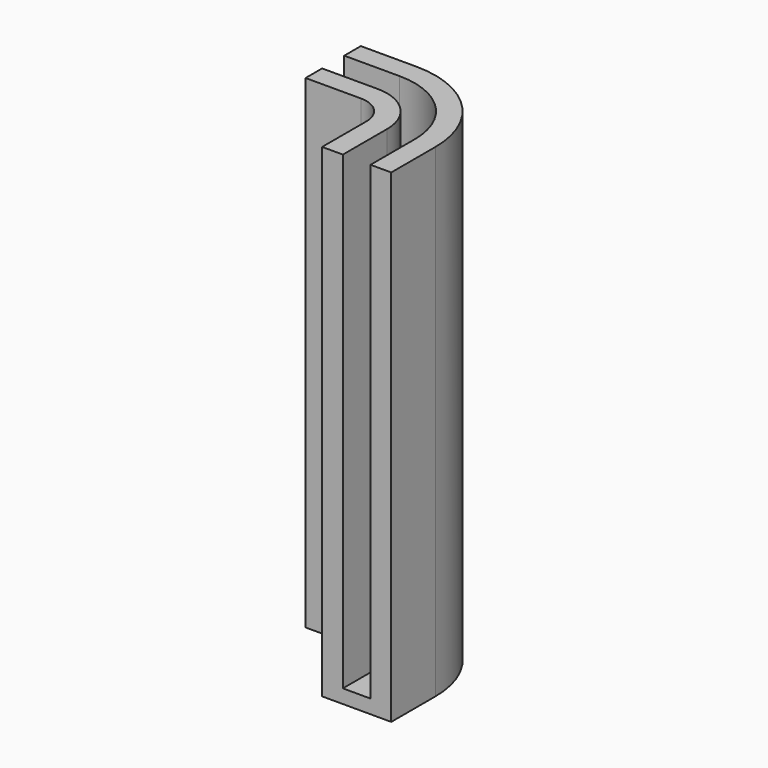
from build123d import *

# Parameters (mm, degrees)
F2_DEPTH = 1
F3_DEPTH = 35


# Not quite as in the source:
# - a feature names something its author has since deleted; it is built from what else it names


with BuildPart() as f2:
    # F1 (on Top) → F2 (new body)
    with BuildSketch(Plane.XY):
        with BuildLine():
            Line((-4, 5.5), (-4, 3.7749172176))
            ThreePointArc((-4, 3.7749172176), (-2.1780674121, 5.0503487353), (0, 5.5))
            Line((0, 5.5), (-4, 5.5))
        make_face()
        with BuildLine():
            ThreePointArc((5.5, 0), (5.0503487353, -2.1780674121), (3.7749172176, -4))
            Line((3.7749172176, -4), (5.5, -4))
            Line((5.5, -4), (5.5, 0))
        make_face()
        with BuildLine():
            Line((-4, 7), (-4, 5.7445626465))
            ThreePointArc((-4, 5.7445626465), (-2.0961943462, 6.6787700412), (0, 7))
            Line((0, 7), (-4, 7))
        make_face()
        with BuildLine():
            ThreePointArc((7, 0), (6.6787700412, -2.0961943462), (5.7445626465, -4))
            Line((5.7445626465, -4), (7, -4))
            Line((7, -4), (7, 0))
        make_face()
        with BuildLine():
            Line((-4, 2), (-2.8722813233, 2))
            ThreePointArc((-2.8722813233, 2), (-1.6201851746, 3.1024184115), (0, 3.5))
            Line((0, 3.5), (-4, 3.5))
            Line((-4, 3.5), (-4, 2))
        make_face()
        with BuildLine():
            ThreePointArc((3.5, 0), (3.1024184115, -1.6201851746), (2, -2.8722813233))
            Line((2, -2.8722813233), (2, -4))
            Line((2, -4), (3.5, -4))
            Line((3.5, -4), (3.5, 0))
        make_face()
        with BuildLine():
            ThreePointArc((0, 2), (1.4142135624, 1.4142135624), (2, 0))
            Line((2, 0), (2, -2.8722813233))
            ThreePointArc((2, -2.8722813233), (3.1024184115, -1.6201851746), (3.5, 0))
            ThreePointArc((3.5, 0), (2.4748737342, 2.4748737342), (0, 3.5))
            ThreePointArc((0, 3.5), (-1.6201851746, 3.1024184115), (-2.8722813233, 2))
            Line((-2.8722813233, 2), (0, 2))
        make_face()
        with BuildLine():
            ThreePointArc((0, 3.5), (2.4748737342, 2.4748737342), (3.5, 0))
            Line((3.5, 0), (3.5, -4))
            Line((3.5, -4), (3.7749172176, -4))
            ThreePointArc((3.7749172176, -4), (5.0503487353, -2.1780674121), (5.5, 0))
            ThreePointArc((5.5, 0), (3.8890872965, 3.8890872965), (0, 5.5))
            ThreePointArc((0, 5.5), (-2.1780674121, 5.0503487353), (-4, 3.7749172176))
            Line((-4, 3.7749172176), (-4, 3.5))
            Line((-4, 3.5), (0, 3.5))
        make_face()
        with BuildLine():
            ThreePointArc((0, 5.5), (3.8890872965, 3.8890872965), (5.5, 0))
            Line((5.5, 0), (5.5, -4))
            Line((5.5, -4), (5.7445626465, -4))
            ThreePointArc((5.7445626465, -4), (6.6787700412, -2.0961943462), (7, 0))
            ThreePointArc((7, 0), (4.9497474683, 4.9497474683), (0, 7))
            ThreePointArc((0, 7), (-2.0961943462, 6.6787700412), (-4, 5.7445626465))
            Line((-4, 5.7445626465), (-4, 5.5))
            Line((-4, 5.5), (0, 5.5))
        make_face()
    extrude(amount=F2_DEPTH)

    # F1 (on Top) → F3 (join)
    with BuildSketch(Plane.XY):
        with BuildLine():
            ThreePointArc((0, 5.5), (3.8890872965, 3.8890872965), (5.5, 0))
            Line((5.5, 0), (5.5, -4))
            Line((5.5, -4), (5.7445626465, -4))
            ThreePointArc((5.7445626465, -4), (6.6787700412, -2.0961943462), (7, 0))
            ThreePointArc((7, 0), (4.9497474683, 4.9497474683), (0, 7))
            ThreePointArc((0, 7), (-2.0961943462, 6.6787700412), (-4, 5.7445626465))
            Line((-4, 5.7445626465), (-4, 5.5))
            Line((-4, 5.5), (0, 5.5))
        make_face()
        with BuildLine():
            Line((-4, 7), (-4, 5.7445626465))
            ThreePointArc((-4, 5.7445626465), (-2.0961943462, 6.6787700412), (0, 7))
            Line((0, 7), (-4, 7))
        make_face()
        with BuildLine():
            ThreePointArc((7, 0), (6.6787700412, -2.0961943462), (5.7445626465, -4))
            Line((5.7445626465, -4), (7, -4))
            Line((7, -4), (7, 0))
        make_face()
        with BuildLine():
            ThreePointArc((3.5, 0), (3.1024184115, -1.6201851746), (2, -2.8722813233))
            Line((2, -2.8722813233), (2, -4))
            Line((2, -4), (3.5, -4))
            Line((3.5, -4), (3.5, 0))
        make_face()
        with BuildLine():
            ThreePointArc((0, 2), (1.4142135624, 1.4142135624), (2, 0))
            Line((2, 0), (2, -2.8722813233))
            ThreePointArc((2, -2.8722813233), (3.1024184115, -1.6201851746), (3.5, 0))
            ThreePointArc((3.5, 0), (2.4748737342, 2.4748737342), (0, 3.5))
            ThreePointArc((0, 3.5), (-1.6201851746, 3.1024184115), (-2.8722813233, 2))
            Line((-2.8722813233, 2), (0, 2))
        make_face()
        with BuildLine():
            Line((-4, 2), (-2.8722813233, 2))
            ThreePointArc((-2.8722813233, 2), (-1.6201851746, 3.1024184115), (0, 3.5))
            Line((0, 3.5), (-4, 3.5))
            Line((-4, 3.5), (-4, 2))
        make_face()
    extrude(amount=F3_DEPTH)


solid = f2.part
